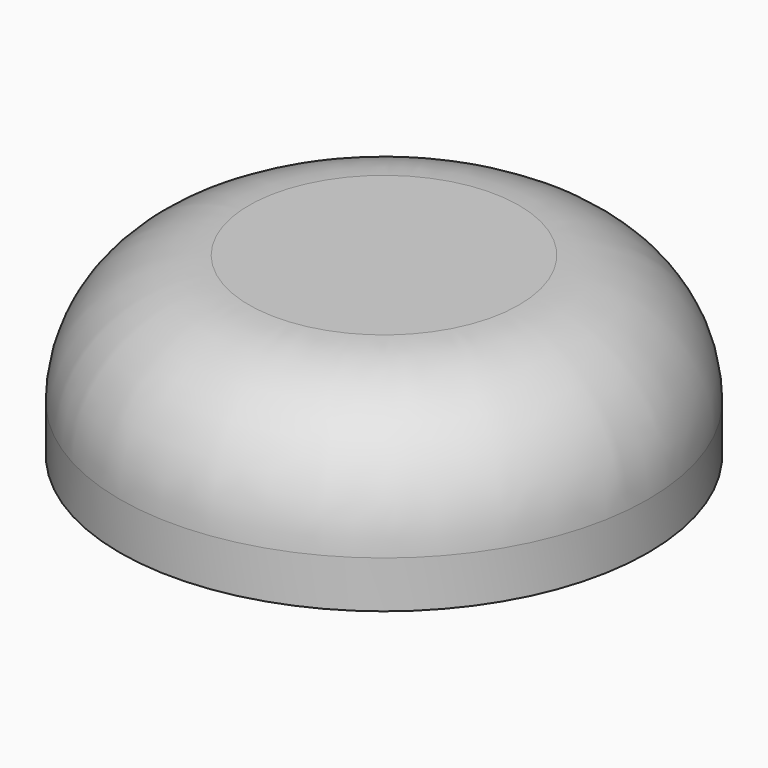
from build123d import *

# Parameters (mm, degrees)
F0_R     = 23.25
F0_W     = 9.8
F0_H     = 9.8
F1_DEPTH = 8
F0_R_2   = 45
F0_R_3   = 29.8
F2_R     = 45
F2_R_2   = 29.8
F3_DEPTH = 22
F4_R     = 21.99999


# Not quite as in the source:
# - a fillet or chamfer is up to 0.001 mm smaller than in the source, because OpenCascade refuses the exact size


with BuildPart() as f1:
    # F0 (on Top) → F1 (new body)
    with BuildSketch(Plane.XY):
        Circle(F0_R)
        Rectangle(F0_W, F0_H, mode=Mode.SUBTRACT)
    extrude(amount=F1_DEPTH)


with BuildPart() as f1b:
    # F0 (on Top) → F1, piece 2 (new body)
    with BuildSketch(Plane.XY):
        Circle(F0_R_2)
        Circle(F0_R_3, mode=Mode.SUBTRACT)
    extrude(amount=F1_DEPTH)


with BuildPart() as f3:
    # F2 (on face) → F3 (new body)
    with BuildSketch(Plane.XY.offset(8)):
        Circle(F2_R)
        Circle(F2_R_2, mode=Mode.SUBTRACT)
        Circle(F2_R_2)
    extrude(amount=F3_DEPTH)

    # F4 (radius 22 in the source; OpenCascade refuses exactly that, so slightly less here)
    f4_edges = [f3.edges().sort_by_distance(p)[0] for p in [
        (-45, 0, 30),
    ]]
    fillet(f4_edges, radius=F4_R)


solid = Compound([f1.part, f1b.part, f3.part])
